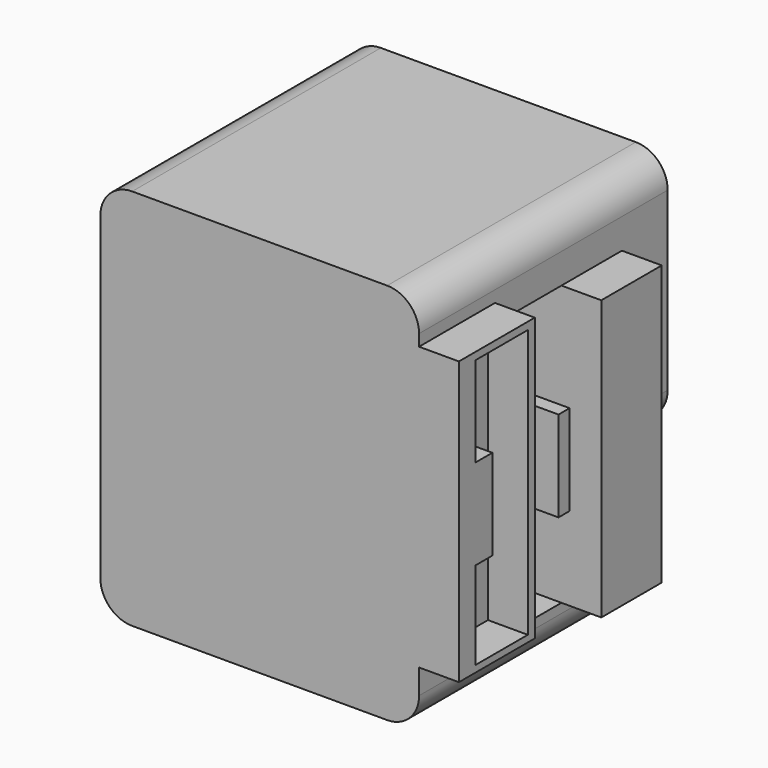
from build123d import *

# Parameters (mm, degrees)
F0_W          = 450
F0_H          = 390
F1_DEPTH      = 480
F2_W          = 94.8382019997
F2_H          = 51.8319234252
F2_H_2        = 77.7373719215
F3_DEPTH      = 50
F4_W          = 42.74310112
F4_H          = 178.9101958275
F4_W_2        = 17.3922628164
F4_H_2        = 113.6361956596
F5_DEPTH      = 400
F6_DEPTH      = 100
F7_W          = 264.5201534033
F7_H          = 243.4637844563
F8_DEPTH      = 25
F9_R          = 40
F10_TEXT_SIZE = 16.6501899162
F11_DEPTH     = 72


# Not quite as in the source:
# - Text() gives the source's letters only with a copy of the font that has no kerning and outlines rounded to 1/6400 em; it was checked with that copy


with BuildPart() as f1:
    # F0 (on Top) → F1 (new body)
    with BuildSketch(Plane.XY):
        with Locations((-225, 195)):
            Rectangle(F0_W, F0_H)
    extrude(amount=F1_DEPTH)

    # F2 (on face) → F3 (cut)
    with BuildSketch(Plane.YZ):
        Polygon((223.3276665211, 402.2626280785), (223.3276665211, 480), (173.6355721951, 480), (173.6355721951, 303.293377161), (173.6355721951, 189.6571815014), (173.6355721951, 0), (223.3276665211, 0), (223.3276665211, 51.8319234252), align=None)
        Polygon((173.6355721951, 303.293377161), (173.6355721951, 480), (0, 480), (0, 425.5047142506), (25.8220676333, 425.5047142506), (119.015738368, 425.5047142506), (119.015738368, 71.1417645216), (25.8220676333, 71.1417645216), (0, 71.1417645216), (0, 0), (173.6355721951, 0), (173.6355721951, 189.6571815014), (156.2433093786, 189.6571815014), (156.2433093786, 303.293377161), align=None)
        Polygon((108.0620363355, 416.2912368774), (25.8220676333, 416.2912368774), (25.8220676333, 303.293377161), (52.4749159813, 303.293377161), (52.4749159813, 189.6571815014), (25.8220676333, 189.6571815014), (25.8220676333, 79.5729458332), (108.0620363355, 79.5729458332), align=None)
        Polygon((390, 0), (390, 480), (318.1658685207, 480), (318.1658685207, 402.2626280785), (318.1658685207, 51.8319234252), (318.1658685207, 0), align=None)
        with Locations((270.7467675209, 25.9159617126)):
            Rectangle(F2_W, F2_H)
        with Locations((270.7467675209, 441.1313140392)):
            Rectangle(F2_W, F2_H_2)
    extrude(amount=-F3_DEPTH, mode=Mode.SUBTRACT)

    # F4 (on face) → F5 (cut)
    with BuildSketch(Plane.YZ.offset(-50)):
        with Locations((368.62844944, 89.4550979137)):
            Rectangle(F4_W, F4_H)
        with Locations((164.9394407868, 246.4752793312)):
            Rectangle(F4_W_2, F4_H_2)
    extrude(amount=-F5_DEPTH, mode=Mode.SUBTRACT)

    # F4 (on face) → F6 (cut)
    with BuildSketch(Plane.YZ.offset(-50)):
        Polygon((156.2433093786, 189.6571815014), (156.2433093786, 51.8319234252), (223.3276665211, 51.8319234252), (223.3276665211, 402.2626280785), (156.2433093786, 402.2626280785), (156.2433093786, 303.293377161), (173.6355721951, 303.293377161), (173.6355721951, 189.6571815014), align=None)
    extrude(amount=-F6_DEPTH, mode=Mode.SUBTRACT)

    # F7 (on face) → F8 (cut)
    with BuildSketch(Plane(origin=(0, 390, 0), x_dir=(-1, 0, 0), z_dir=(0, 1, 0))):
        with Locations((251.6159191728, 300.6420880556)):
            Rectangle(F7_W, F7_H)
    extrude(amount=-F8_DEPTH, mode=Mode.SUBTRACT)

    # F9
    f9_edges = [f1.edges().sort_by_distance(p)[0] for p in [
        (-50, 195, 480),
        (-50, 368.628449, 178.910196),
        (-50, 173.628449, 0),
        (-450, 173.628449, 0),
        (-450, 368.628449, 178.910196),
        (-450, 195, 480),
    ]]
    fillet(f9_edges, radius=F9_R)

    # F10 (on face) → F11 (join)
    with BuildSketch(Plane(origin=(0, 318.1658685207, 0), x_dir=(-1, 0, 0), z_dir=(0, 1, 0))):
        with Locations((220, 448.0118632603)):
            Text('Canon', F10_TEXT_SIZE, font='Open Sans', text_align=(TextAlign.LEFT, TextAlign.BOTTOM))
    extrude(amount=F11_DEPTH)


solid = f1.part
